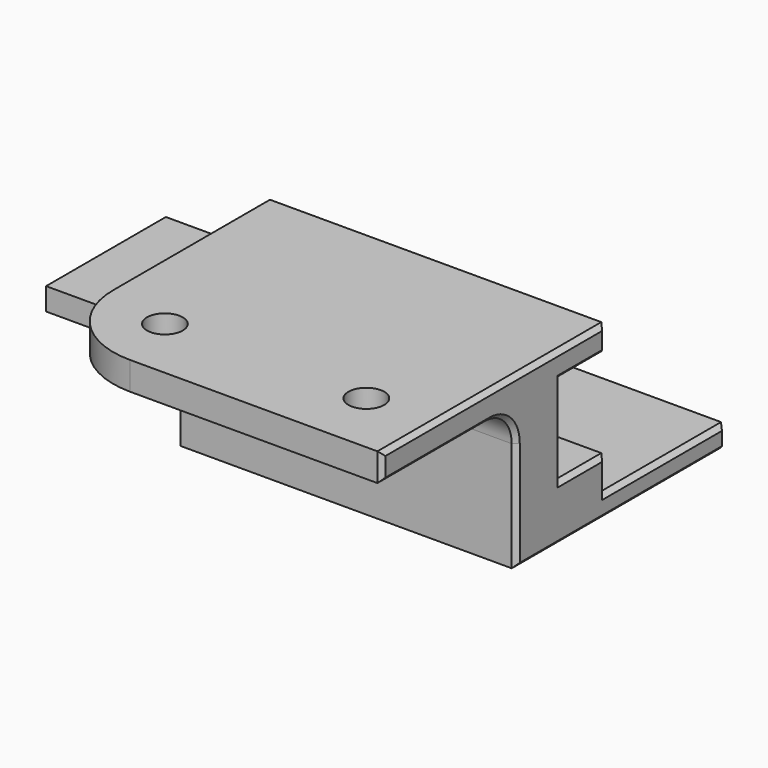
from build123d import *

# Parameters (mm, degrees)
F0_W     = 13.375
F0_H     = 2
F1_DEPTH = 25
F2_R     = 1.75
F3_DEPTH = 2
F5_DEPTH = 30
F6_W     = 5
F6_H     = 8
F7_DEPTH = 50.001
F8_R     = 1.6
F9_DEPTH = 2.5
F10_R    = 7.5
F11_R    = 3
F12_R    = 2
F13_SIZE = 0.4


with BuildPart() as f1:
    # F0 (on Right) → F1 (new body, symmetric)
    with BuildSketch(Plane.YZ):
        with Locations((6.6875, 1)):
            Rectangle(F0_W, F0_H)
    extrude(amount=F1_DEPTH, both=True)

    # F2 (on face) → F3 (cut, through all)
    with BuildSketch(Plane.XY.offset(2)):
        with Locations((-13, 4)):
            Circle(F2_R)
        with Locations((13, 4)):
            Circle(F2_R)
    extrude(amount=-F3_DEPTH, mode=Mode.SUBTRACT)

    # F4 (on face) → F5 (join)
    with BuildSketch(Plane.YZ.offset(25)):
        Polygon((-10, 0), (0, 0), (0, 15.3), (-25, 15.3), (-25, 12.8), (-10, 12.8), align=None)
    extrude(amount=-F5_DEPTH)

    # F6 (on face) → F7 (cut, through all)
    with BuildSketch(Plane.YZ.offset(25)):
        with Locations((-2.5, 9)):
            Rectangle(F6_W, F6_H)
    extrude(amount=-F7_DEPTH, mode=Mode.SUBTRACT)

    # F8 (on face) → F9 (cut, through all)
    with BuildSketch(Plane(origin=(0, 0, 12.8), x_dir=(1, 0, 0), z_dir=(0, 0, -1))):
        with Locations((1, 19.235)):
            Circle(F8_R)
        with Locations((19, 19.235)):
            Circle(F8_R)
    extrude(amount=-F9_DEPTH, mode=Mode.SUBTRACT)

    # F10
    f10_edges = [f1.edges().sort_by_distance(p)[0] for p in [
        (-5, -25, 14.05),
    ]]
    fillet(f10_edges, radius=F10_R)

    # F11
    f11_edges = [f1.edges().sort_by_distance(p)[0] for p in [
        (10, -10, 12.8),
    ]]
    fillet(f11_edges, radius=F11_R)

    # F12
    f12_edges = [f1.edges().sort_by_distance(p)[0] for p in [
        (-5, 0, 1),
    ]]
    fillet(f12_edges, radius=F12_R)

    # F13
    f13_edges = [f1.edges().sort_by_distance(p)[0] for p in [
        (25, -10, 4.9),
        (25, -10.87868, 11.92132),
        (25, 1.6875, 0),
        (25, -19, 12.8),
        (25, 13.375, 1),
        (25, -25, 14.05),
        (25, 6.6875, 2),
        (25, -12.5, 15.3),
        (25, 0, 3.5),
        (25, 0, 14.15),
        (25, -2.5, 5),
        (25, -2.5, 13),
        (25, -5, 9),
    ]]
    chamfer(f13_edges, length=F13_SIZE)


solid = f1.part
